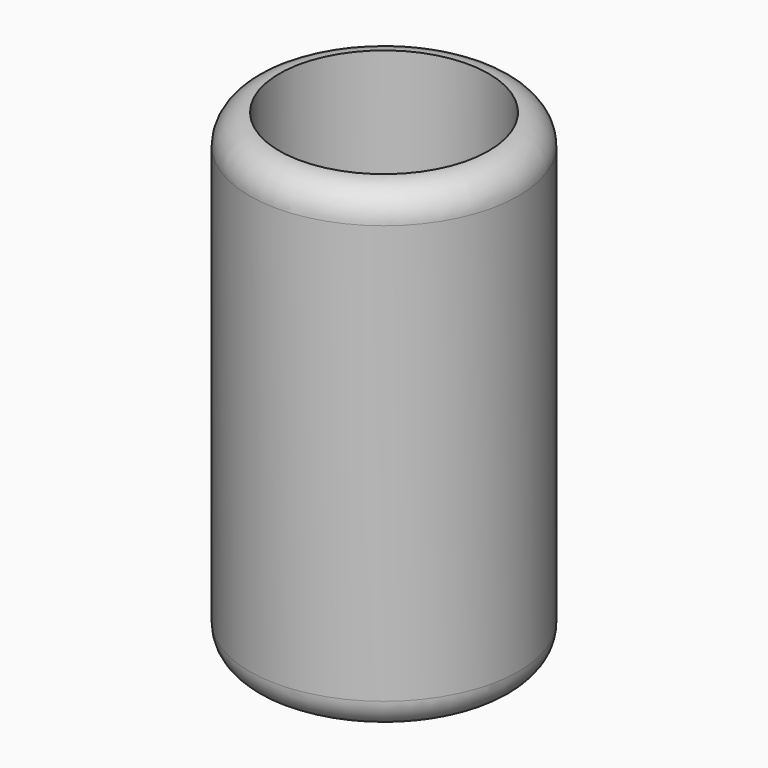
from build123d import *

# Parameters (mm, degrees)
F0_R     = 22.5
F0_R_2   = 17.5
F1_DEPTH = 80
F2_R     = 4.99999


# Not quite as in the source:
# - a fillet or chamfer is up to 0.001 mm smaller than in the source, because OpenCascade refuses the exact size


with BuildPart() as f1:
    # F0 (on Top) → F1 (new body)
    with BuildSketch(Plane.XY):
        Circle(F0_R)
        Circle(F0_R_2, mode=Mode.SUBTRACT)
    extrude(amount=F1_DEPTH)

    # F2 (radius 5 in the source; OpenCascade refuses exactly that, so slightly less here)
    f2_edges = [f1.edges().sort_by_distance(p)[0] for p in [
        (-22.5, 0, 80),
        (-22.5, 0, 0),
    ]]
    fillet(f2_edges, radius=F2_R)


solid = f1.part
